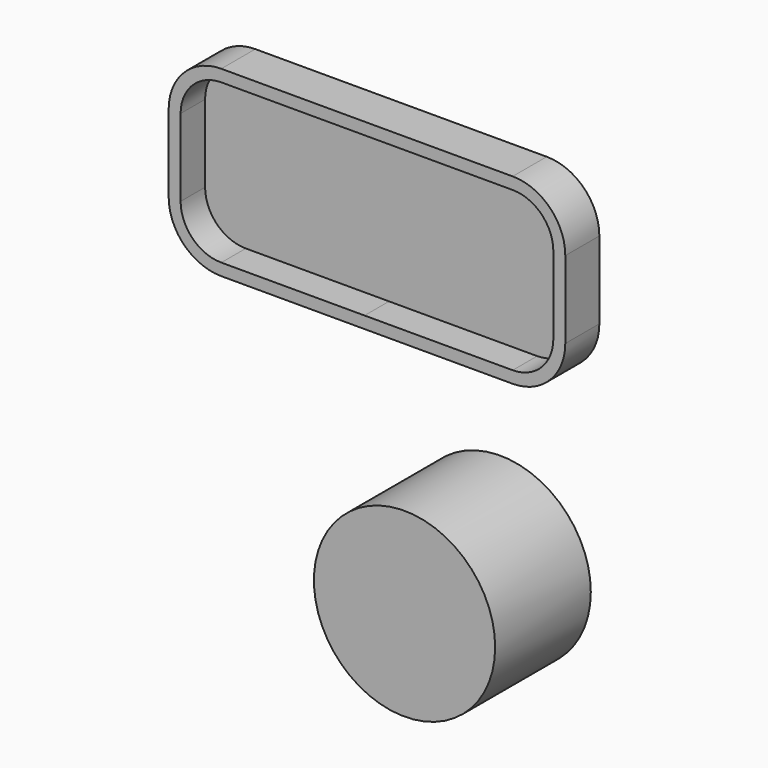
from build123d import *

# Parameters (mm, degrees)
F1_DEPTH = 8.9
F2_T     = -2.5
F3_R     = 18.9471893283
F4_DEPTH = 25


# Not quite as in the source:
# - ends of sketch curves that miss each other by under 0.0002 mm in the source are joined


with BuildPart() as f1:
    # F0 (on Front) → F1 (new body)
    with BuildSketch(Plane.XZ):
        with BuildLine():
            Line((-21.2359558791, 45.1264046133), (-51.1910132468, 45.1264046133))
            ThreePointArc((-51.1910132468, 45.1264046133), (-58.9691878398, 41.9045792063), (-62.1910132468, 34.1264046133))
            Line((-62.1910132468, 34.1264046133), (-62.1910132468, 17.9522452541))
            ThreePointArc((-62.1910132468, 17.9522452541), (-58.9691878398, 10.174070661), (-51.1910132468, 6.9522452541))
            Line((-51.1910132468, 6.9522452541), (-21.2359558791, 6.9522452541))
            Line((-21.2359558791, 6.9522452541), (9.7303389907, 6.952248048))
            ThreePointArc((9.7303389907, 6.952248048), (17.5085135837, 10.174073455), (20.7303389907, 17.952248048))
            Line((20.7303389907, 17.952248048), (20.7303389907, 34.1264046133))
            ThreePointArc((20.7303389907, 34.1264046133), (17.5085135837, 41.9045792063), (9.7303389907, 45.1264046133))
            Line((9.7303389907, 45.1264046133), (-21.2359558791, 45.1264046133))
        make_face()
    extrude(amount=F1_DEPTH)

    # F2
    f2_openings = [f1.faces().sort_by_distance(p)[0] for p in [
        (-20.730338, -8.9, 26.039325),
    ]]
    offset(amount=F2_T, openings=f2_openings)


with BuildPart() as f4:
    # F3 (on Front) → F4 (new body)
    with BuildSketch(Plane.XZ):
        with Locations((0, -31.9803394377)):
            Circle(F3_R)
    extrude(amount=F4_DEPTH)


solid = Compound([f1.part, f4.part])
